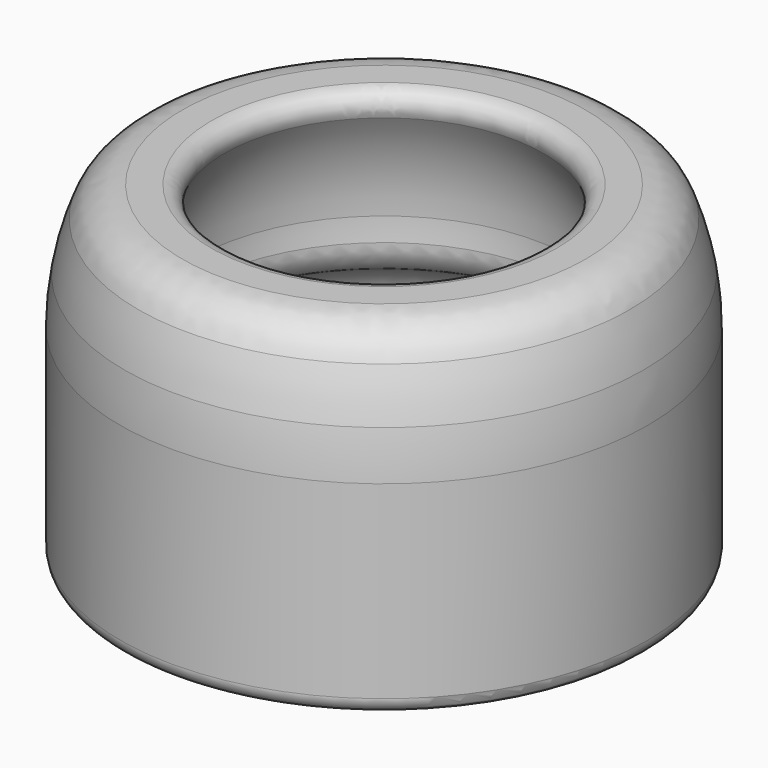
from build123d import *

# Parameters (mm, degrees)
F2_R   = 2
F5_R   = 1
F5_2_R = 1
F6_R   = 3


with BuildPart() as f1:
    # F0 (on Front) → F1 (revolve)
    with BuildSketch(Plane.XZ):
        with BuildLine():
            ThreePointArc((11.5623058987, -3.211398808), (14.7224318643, -8.5), (8.5623058987, -8.4075512307))
            ThreePointArc((8.5623058987, -8.4075512307), (4.6427031583, -11.0655007742), (0, -12))
            Line((0, -12), (0, -13))
            Line((0, -13), (16.7463987921, -13))
            Line((16.7463987921, -13), (16.7463987921, 0))
            ThreePointArc((16.7463987921, 0), (16.6785348586, 1.5061034078), (16.4754930884, 3))
            Line((16.4754930884, 3), (13.5, 3))
            Line((13.5, 3), (13.5, 0))
            Line((13.5, 0), (12, 0))
            ThreePointArc((12, 0), (11.8900729768, -1.6205445404), (11.5623058987, -3.211398808))
        make_face()
    revolve(axis=Axis((0, 0, -1.5362007543), (0, 0, 1)))

    # F2
    f2_edges = [f1.edges().sort_by_distance(p)[0] for p in [
        (-8.562306, 0, -8.407551),
        (-11.562306, 0, -3.211399),
    ]]
    fillet(f2_edges, radius=F2_R)

    # F5
    f5_edges = [f1.edges().sort_by_distance(p)[0] for p in [
        (-16.746399, 0, -13),
    ]]
    fillet(f5_edges, radius=F5_R)


with BuildPart() as f4:
    # F3 (on Front) → F4 (revolve)
    with BuildSketch(Plane.XZ):
        with BuildLine():
            ThreePointArc((8.94427191, 8), (11.2100683076, 4.2818650773), (12, 0))
            Line((12, 0), (13.5, 0))
            Line((13.5, 0), (13.5, 3))
            Line((13.5, 3), (16.4754930884, 3))
            ThreePointArc((16.4754930884, 3), (15.7928579879, 5.5702342032), (14.7119635843, 8))
            Line((14.7119635843, 8), (8.94427191, 8))
        make_face()
    revolve(axis=Axis((0, 0, -1.5362007543), (0, 0, 1)))

    # F5#2
    f5_2_edges = [f4.edges().sort_by_distance(p)[0] for p in [
        (-8.944272, 0, 8),
    ]]
    fillet(f5_2_edges, radius=F5_2_R)

    # F6
    f6_edges = [f4.edges().sort_by_distance(p)[0] for p in [
        (-14.711964, 0, 8),
    ]]
    fillet(f6_edges, radius=F6_R)


solid = Compound([f1.part, f4.part])
